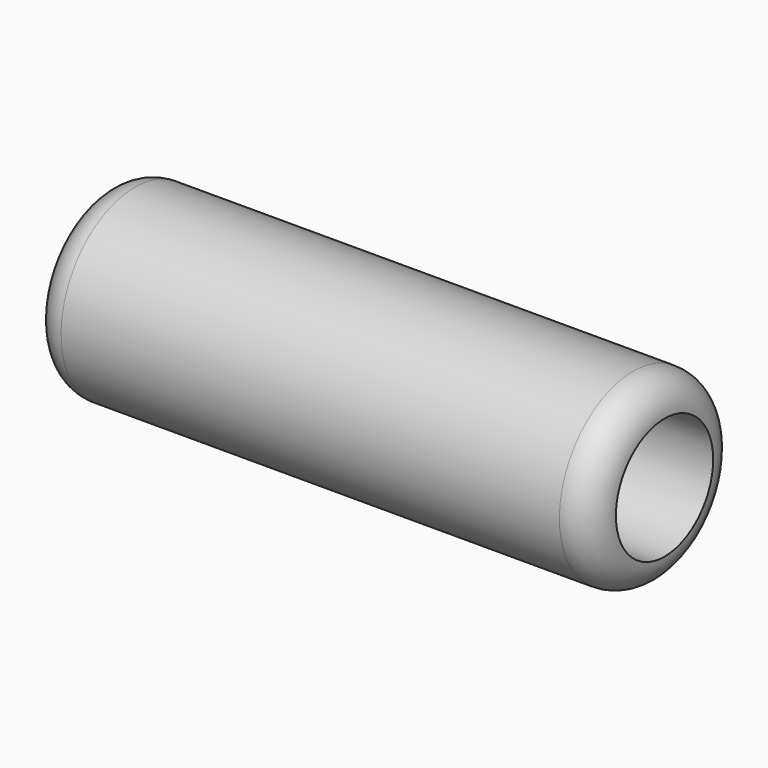
from build123d import *

# Parameters (mm, degrees)
F2_R = 6.34999


# Not quite as in the source:
# - a fillet or chamfer is up to 0.001 mm smaller than in the source, because OpenCascade refuses the exact size


with BuildPart() as f1:
    # F0 (on Front) → F1 (revolve)
    with BuildSketch(Plane.XZ):
        Polygon((-109.2541576196, -73.9613701678), (-113.2165576196, -73.9613701678), (-113.2165576196, -91.4238701678), (0.2960423804, -91.4238701678), (0.2960423804, -85.0738701678), (-109.2541576196, -85.0738701678), align=None)
    revolve(axis=Axis((-12.7451103181, 0, -72.7707451678), (1, 0, 0)))

    # F2 (radius 6.35 in the source; OpenCascade refuses exactly that, so slightly less here)
    f2_edges = [f1.edges().sort_by_distance(p)[0] for p in [
        (0.296042, 0, -54.11762),
        (-113.216558, 0, -54.11762),
    ]]
    fillet(f2_edges, radius=F2_R)


solid = f1.part
